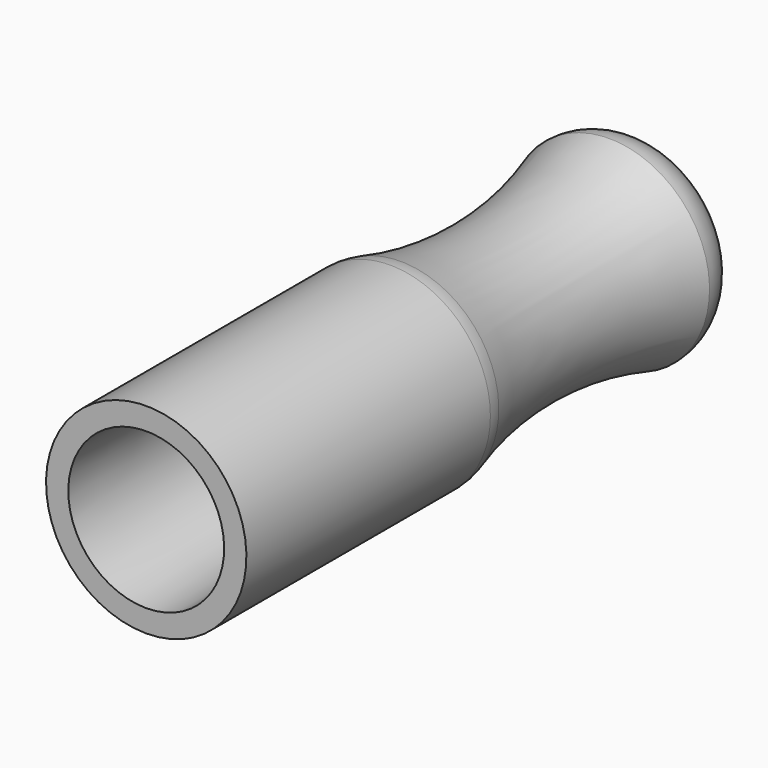
from build123d import *

# Parameters (mm, degrees)
F2_R = 1.99999
F3_R = 2


# Not quite as in the source:
# - a fillet or chamfer is up to 0.001 mm smaller than in the source, because OpenCascade refuses the exact size


with BuildPart() as f1:
    # F0 (on Right) → F1 (revolve)
    with BuildSketch(Plane.YZ):
        with BuildLine():
            Line((-2, -4.5), (0, -4.5))
            Line((0, -4.5), (0, -2))
            Line((0, -2), (-14.007930782, -2.2))
            Line((-14.007930782, -2.2), (-14.007930782, -3))
            Line((-14.007930782, -3), (-28, -3.5))
            Line((-28, -3.5), (-28, -4.5))
            Line((-28, -4.5), (-14, -4.5))
            ThreePointArc((-14, -4.5), (-8, -3.5651046907), (-2, -4.5))
        make_face()
    revolve(axis=Axis((0, -15.99, 0), (0, -1, 0)))

    # F2 (radius 2 in the source; OpenCascade refuses exactly that, so slightly less here)
    f2_edges = [f1.edges().sort_by_distance(p)[0] for p in [
        (0, 0, 4.5),
    ]]
    fillet(f2_edges, radius=F2_R)

    # F3
    f3_edges = [f1.edges().sort_by_distance(p)[0] for p in [
        (0, -14, 4.5),
    ]]
    fillet(f3_edges, radius=F3_R)


solid = f1.part
